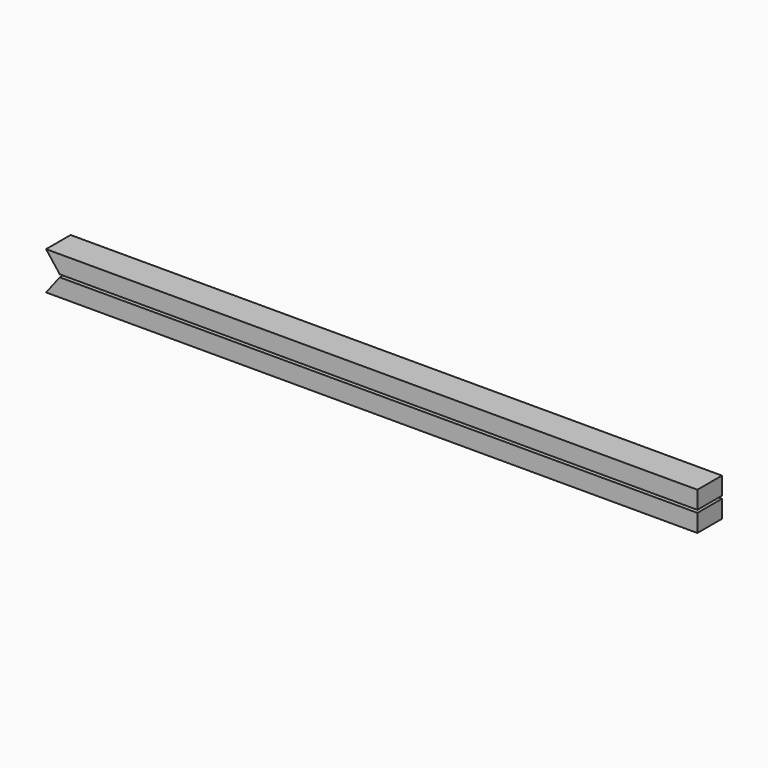
from build123d import *

# Parameters (mm, degrees)
F1_DEPTH = 3.175


# Not quite as in the source:
# - a feature names something its author has since deleted; it is built from what else it names


with BuildPart() as f1:
    # F0 (on Front) → F1 (new body)
    with BuildSketch(Plane.XZ):
        Polygon((-6.1159002899, -0.1391640983), (-13.6670420062, -0.1391640983), (-41.0246514305, -0.1391640983), (-52.8478002203, -0.1391640983), (-54.263135106, -1.9746770844), (13.2233296217, -1.9746770844), (13.2233296217, -0.1391640983), align=None)
    extrude(amount=F1_DEPTH)


with BuildPart() as f1b:
    # F0 (on Front) → F1, piece 2 (new body)
    with BuildSketch(Plane.XZ):
        Polygon((13.2233296217, 1.9746770844), (-54.263135106, 1.9746770844), (-52.8478002203, 0.1391640983), (-41.0246514305, 0.1391640983), (-13.6670420062, 0.1391640983), (-6.1159002899, 0.1391640983), (13.2233296217, 0.1391640983), align=None)
    extrude(amount=F1_DEPTH)


solid = Compound([f1.part, f1b.part])
